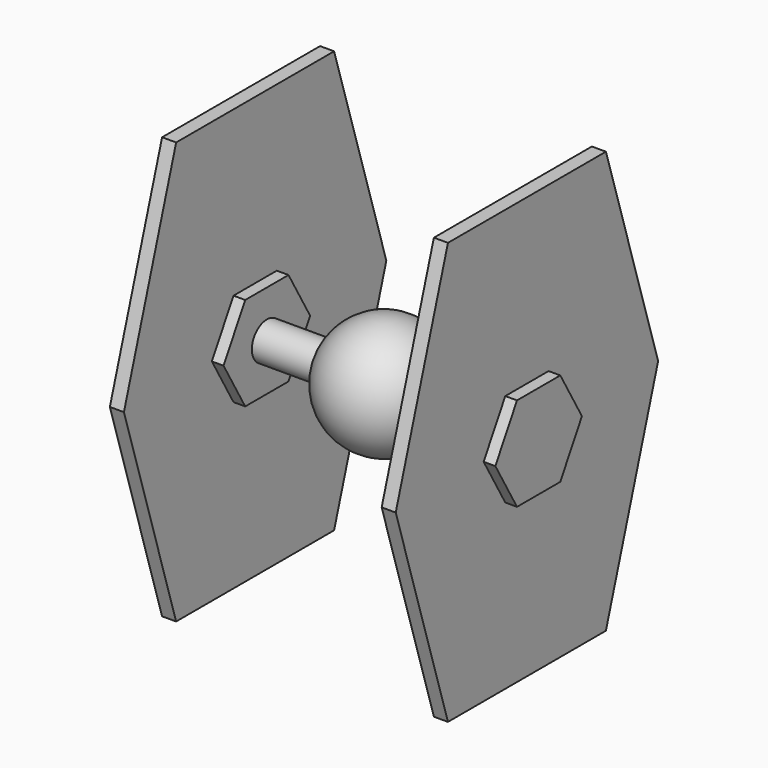
from build123d import *

# Parameters (mm, degrees)
F2_R          = 8
F3_DEPTH      = 55
F5_DEPTH      = 6
F7_DEPTH      = 5
F7_DEPTH_BACK = 11


# Not quite as in the source:
# - a pattern or mirror of a feature is missing from the dataset's text; its kind, count and spacing are read off the source's solid


with BuildPart() as f1:
    # F0 (on Front) → F1 (revolve)
    with BuildSketch(Plane.XZ):
        with BuildLine():
            Line((0, -25), (0, 25))
            ThreePointArc((0, 25), (-25, 0), (0, -25))
        make_face()
    revolve(axis=Axis((0, 0, 0), (0, 0, -1)))

    # F2 (on Right) → F3 (join)
    with BuildSketch(Plane.YZ):
        Circle(F2_R)
    f3 = extrude(amount=F3_DEPTH)

    # F3_copies: F3 across plane
    add(f3.mirror(Plane(origin=(0, 0, 0), x_dir=(0, 0, -1), z_dir=(-1, 0, 0))))

    # F4 (on face) → F5 (join)
    with BuildSketch(Plane.YZ.offset(55)):
        Polygon((-42.1359225246, 90), (-70, 0), (-42.1359225246, -90), (42.1359225246, -90), (70, 0), (42.1359225246, 90), align=None)
    f5 = extrude(amount=F5_DEPTH)

    # F5_copies: F5 across plane
    add(f5.mirror(Plane(origin=(0, 0, 0), x_dir=(0, 0, -1), z_dir=(-1, 0, 0))))

    # F6 (on face) → F7 (join, two sides)
    with BuildSketch(Plane.YZ.offset(61)) as f7_sk:
        Polygon((-11.5470053838, -20), (11.5470053838, -20), (23.0940107676, 0), (11.5470053838, 20), (-11.5470053838, 20), (-23.0940107676, 0), align=None)
    f7 = extrude(amount=F7_DEPTH) + extrude(f7_sk.sketch, amount=-F7_DEPTH_BACK)

    # F7_copies: F7 across plane
    add(f7.mirror(Plane(origin=(0, 0, 0), x_dir=(0, 0, -1), z_dir=(-1, 0, 0))))


solid = f1.part
